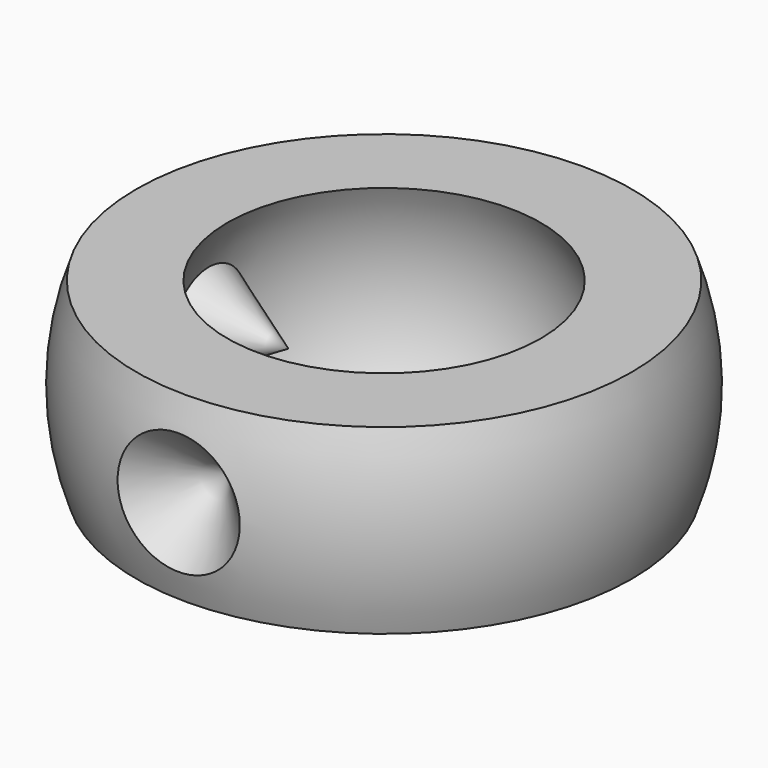
from build123d import *


# Not quite as in the source:
# - a pattern or mirror of a feature is missing from the dataset's text; its kind, count and spacing are read off the source's solid


with BuildPart() as f1:
    # F0 (on Front) → F1 (revolve)
    with BuildSketch(Plane.XZ):
        with BuildLine():
            Line((27.2213151776, 10), (17.2213151776, 10))
            ThreePointArc((17.2213151776, 10), (19.9141581908, 0), (17.2213151776, -10))
            Line((17.2213151776, -10), (27.2213151776, -10))
            Line((27.2213151776, -10), (27.2213151776, 10))
        make_face()
        with BuildLine():
            ThreePointArc((27.2213151776, -10), (29, 0), (27.2213151776, 10))
            Line((27.2213151776, 10), (27.2213151776, -10))
        make_face()
    revolve(axis=Axis((0, 0, -0.0082536135), (0, 0, -1)))

    # F2 (on Top) → F3 (revolve, cut)
    with BuildSketch(Plane.XY):
        Polygon((0, 30.5), (0, 21.5), (9, 30.5), align=None)
    f3 = revolve(axis=Axis((0, 26, 0), (0, -1, 0)), mode=Mode.SUBTRACT)

    # F3_copies: F3 across plane
    add(f3.mirror(Plane(origin=(0, 0, 0), x_dir=(0, 0, -1), z_dir=(0, -1, 0))), mode=Mode.SUBTRACT)

    # F4 (on Top) → F5 (revolve)
    with BuildSketch(Plane.XY):
        Polygon((-10.5096189432, 0), (-23.5, 7.5), (-23.5, 0), align=None)
    f5 = revolve(axis=Axis((-17.0048094716, 0, 0), (-1, 0, 0)))

    # F5_copies: F5 across plane
    add(f5.mirror(Plane(origin=(0, 0, 0), x_dir=(0, 0, 1), z_dir=(1, 0, 0))))


solid = f1.part
